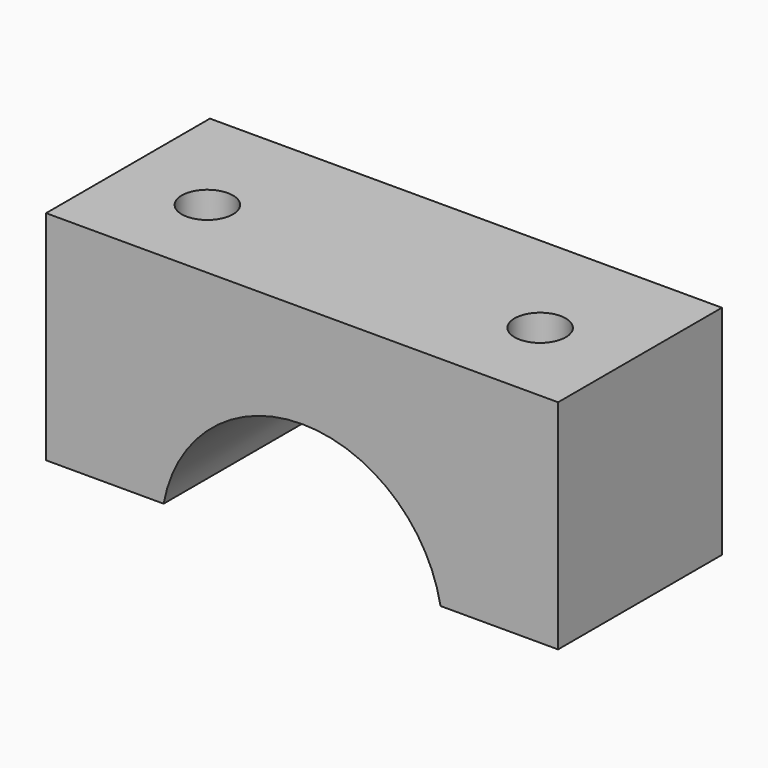
from build123d import *

# Parameters (mm, degrees)
F1_DEPTH = 16
F3_D     = 4


# Not quite as in the source:
# - a feature of the source that left no trace in its solid (it failed there, or was rolled back) is left out
# - the program builds the solid bodies; features that only make, move or delete a surface that nothing else refers to are left out


with BuildPart() as f1:
    # F0 (on Front) → F1 (new body)
    with BuildSketch(Plane.XZ):
        with BuildLine():
            ThreePointArc((-10.8166538264, 0), (0, 9), (10.8166538264, 0))
            Line((10.8166538264, 0), (20, 0))
            Line((20, 0), (20, 17))
            Line((20, 17), (-20, 17))
            Line((-20, 17), (-20, 0))
            Line((-20, 0), (-10.8166538264, 0))
        make_face()
    extrude(amount=F1_DEPTH)

    # F3 (through all)
    with Locations(Plane.XY.offset(17)):
        with Locations((13, -9), (-13, -9)):
            Hole(F3_D / 2)


solid = f1.part
